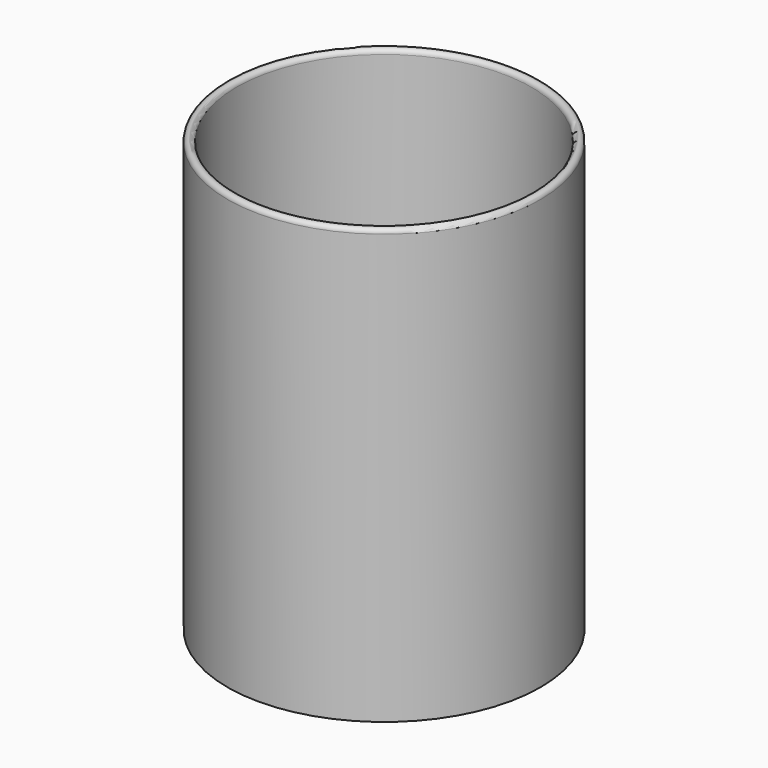
from build123d import *

# Parameters (mm, degrees)
F0_R     = 35
F1_DEPTH = 100
F2_T     = -2
F5_R     = 10


# Not quite as in the source:
# - a fillet or chamfer that OpenCascade refuses, or shapes differently, is made with other operations: its cross-section is extruded or revolved along the edge and cut away or added


with BuildPart() as f1:
    # F0 (on Top) → F1 (new body)
    with BuildSketch(Plane.XY):
        Circle(F0_R)
    extrude(amount=F1_DEPTH)

    # F2
    f2_openings = [f1.faces().sort_by_distance(p)[0] for p in [
        (0, 0, 100),
    ]]
    offset(amount=F2_T, openings=f2_openings)

    # F3: fillet of radius 5 on 1 edges, made by hand

    # F3_s1 → F3_t2 (revolve, cut)
    with BuildSketch(Plane.XZ):
        with BuildLine():
            ThreePointArc((35, 96), (34.472135955, 98.2360679775), (33, 100))
            Line((33, 100), (35, 100))
            Line((35, 100), (35, 96))
        make_face()
    revolve(axis=Axis((0, 0, 100), (0, 0, 1)), mode=Mode.SUBTRACT)

    # F4: fillet of radius 1 on 1 edges, made by hand

    # F4_s1 → F4_t2 (revolve, cut)
    with BuildSketch(Plane.XZ):
        with BuildLine():
            ThreePointArc((35, 96.0000100581), (33.9999989942, 97.0000080465), (33, 96.0000080465))
            Line((33, 96.0000080465), (33, 100))
            ThreePointArc((33, 100), (34.4721337059, 98.2360724756), (35, 96.0000100581))
        make_face()
    revolve(axis=Axis((0, 0, 100), (0, 0, 1)), mode=Mode.SUBTRACT)

    # F5
    f5_edges = [f1.edges().sort_by_distance(p)[0] for p in [
        (-33, 0, 2),
    ]]
    fillet(f5_edges, radius=F5_R)


solid = f1.part
